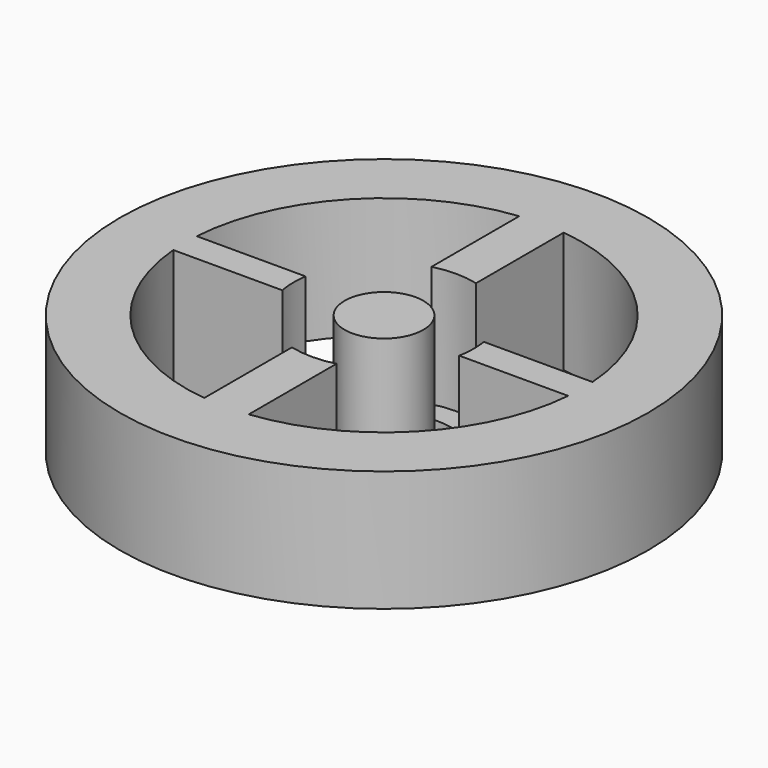
from build123d import *

# Parameters (mm, degrees)
F0_R     = 55.4446440976
F1_DEPTH = 25.4
F2_DEPTH = 25.4
F0_R_2   = 14.2471113664
F3_DEPTH = 7.112
F0_R_3   = 8.2640856971
F4_DEPTH = 25.4


# Not quite as in the source:
# - a feature names something its author has since deleted; it is built from what else it names


with BuildPart() as f1:
    # F0 (on Top) → F1 (new body)
    with BuildSketch(Plane.XY):
        Circle(F0_R)
        with BuildLine():
            ThreePointArc((4.6694431101, 41.3246424597), (30.0430645384, 28.7566348262), (41.4893209282, 2.8576252906))
            ThreePointArc((41.4893209282, 2.8576252906), (41.5630346864, 1.4296576644), (41.5876156251, 0))
            ThreePointArc((41.5876156251, 0), (41.551042786, -1.743736442), (41.4413885942, -3.4844059424))
            ThreePointArc((41.4413885942, -3.4844059424), (29.8248734287, -28.9828690496), (4.6694431101, -41.3246424597))
            ThreePointArc((4.6694431101, -41.3246424597), (0, -41.5876156251), (-4.6694431101, -41.3246424597))
            ThreePointArc((-4.6694431101, -41.3246424597), (-29.8248734287, -28.9828690496), (-41.4413885942, -3.4844059424))
            ThreePointArc((-41.4413885942, -3.4844059424), (-41.5859924727, -0.3674281517), (-41.496486252, 2.7516180913))
            ThreePointArc((-41.496486252, 2.7516180913), (-30.0797741132, 28.7182339757), (-4.6694431101, 41.3246424597))
            ThreePointArc((-4.6694431101, 41.3246424597), (0, 41.5876156251), (4.6694431101, 41.3246424597))
        make_face(mode=Mode.SUBTRACT)
    extrude(amount=F1_DEPTH)

    # F0 (on Top) → F2 (join)
    with BuildSketch(Plane.XY):
        Circle(F0_R)
        with BuildLine():
            ThreePointArc((4.6694431101, 41.3246424597), (30.0430645384, 28.7566348262), (41.4893209282, 2.8576252906))
            ThreePointArc((41.4893209282, 2.8576252906), (41.5630346864, 1.4296576644), (41.5876156251, 0))
            ThreePointArc((41.5876156251, 0), (41.551042786, -1.743736442), (41.4413885942, -3.4844059424))
            ThreePointArc((41.4413885942, -3.4844059424), (29.8248734287, -28.9828690496), (4.6694431101, -41.3246424597))
            ThreePointArc((4.6694431101, -41.3246424597), (0, -41.5876156251), (-4.6694431101, -41.3246424597))
            ThreePointArc((-4.6694431101, -41.3246424597), (-29.8248734287, -28.9828690496), (-41.4413885942, -3.4844059424))
            ThreePointArc((-41.4413885942, -3.4844059424), (-41.5859924727, -0.3674281517), (-41.496486252, 2.7516180913))
            ThreePointArc((-41.496486252, 2.7516180913), (-30.0797741132, 28.7182339757), (-4.6694431101, 41.3246424597))
            ThreePointArc((-4.6694431101, 41.3246424597), (0, 41.5876156251), (4.6694431101, 41.3246424597))
        make_face(mode=Mode.SUBTRACT)
        with BuildLine():
            ThreePointArc((-4.6694431101, 18.3096772012), (0, 18.895713222), (4.6694431101, 18.3096772012))
            Line((4.6694431101, 18.3096772012), (4.6694431101, 41.3246424597))
            ThreePointArc((4.6694431101, 41.3246424597), (0, 41.5876156251), (-4.6694431101, 41.3246424597))
            Line((-4.6694431101, 41.3246424597), (-4.6694431101, 18.3096772012))
        make_face()
        with BuildLine():
            ThreePointArc((-18.5716691064, -3.4844059424), (-18.8920611509, -0.3714884108), (-18.6942926063, 2.7516180913))
            Line((-18.6942926063, 2.7516180913), (-41.496486252, 2.7516180913))
            ThreePointArc((-41.496486252, 2.7516180913), (-41.5859924727, -0.3674281517), (-41.4413885942, -3.4844059424))
            Line((-41.4413885942, -3.4844059424), (-18.5716691064, -3.4844059424))
        make_face()
        with BuildLine():
            Line((4.6694431101, -41.3246424597), (4.6694431101, -18.3096772012))
            ThreePointArc((4.6694431101, -18.3096772012), (0, -18.895713222), (-4.6694431101, -18.3096772012))
            Line((-4.6694431101, -18.3096772012), (-4.6694431101, -41.3246424597))
            ThreePointArc((-4.6694431101, -41.3246424597), (0, -41.5876156251), (4.6694431101, -41.3246424597))
        make_face()
        with BuildLine():
            ThreePointArc((18.6783820463, 2.8576252906), (18.8413020883, 1.4329388631), (18.895713222, 0))
            ThreePointArc((18.895713222, 0), (18.8145277865, -1.7497206463), (18.5716691064, -3.4844059424))
            Line((18.5716691064, -3.4844059424), (41.4413885942, -3.4844059424))
            ThreePointArc((41.4413885942, -3.4844059424), (41.551042786, -1.743736442), (41.5876156251, 0))
            ThreePointArc((41.5876156251, 0), (41.5630346864, 1.4296576644), (41.4893209282, 2.8576252906))
            Line((41.4893209282, 2.8576252906), (18.6783820463, 2.8576252906))
        make_face()
    extrude(amount=F2_DEPTH)


with BuildPart() as f3:
    # F0 (on Top) → F3 (new body)
    with BuildSketch(Plane.XY):
        with BuildLine():
            Line((41.4413885942, -3.4844059424), (18.5716691064, -3.4844059424))
            ThreePointArc((18.5716691064, -3.4844059424), (13.7834861787, -12.925304133), (4.6694431101, -18.3096772012))
            Line((4.6694431101, -18.3096772012), (4.6694431101, -41.3246424597))
            ThreePointArc((4.6694431101, -41.3246424597), (29.8248734287, -28.9828690496), (41.4413885942, -3.4844059424))
        make_face()
        with BuildLine():
            ThreePointArc((18.5716691064, -3.4844059424), (18.8145277865, -1.7497206463), (18.895713222, 0))
            ThreePointArc((18.895713222, 0), (18.8413020883, 1.4329388631), (18.6783820463, 2.8576252906))
            ThreePointArc((18.6783820463, 2.8576252906), (13.9989896759, 12.6915824949), (4.6694431101, 18.3096772012))
            ThreePointArc((4.6694431101, 18.3096772012), (0, 18.895713222), (-4.6694431101, 18.3096772012))
            ThreePointArc((-4.6694431101, 18.3096772012), (-14.0349327563, 12.6518236115), (-18.6942926063, 2.7516180913))
            ThreePointArc((-18.6942926063, 2.7516180913), (-18.8920611509, -0.3714884108), (-18.5716691064, -3.4844059424))
            ThreePointArc((-18.5716691064, -3.4844059424), (-13.7834861787, -12.925304133), (-4.6694431101, -18.3096772012))
            ThreePointArc((-4.6694431101, -18.3096772012), (0, -18.895713222), (4.6694431101, -18.3096772012))
            ThreePointArc((4.6694431101, -18.3096772012), (13.7834861787, -12.925304133), (18.5716691064, -3.4844059424))
        make_face()
        Circle(F0_R_2, mode=Mode.SUBTRACT)
    extrude(amount=-F3_DEPTH)


with BuildPart() as f4:
    # F0 (on Top) → F4 (new body)
    with BuildSketch(Plane.XY):
        Circle(F0_R_3)
    extrude(amount=F4_DEPTH)


solid = Compound([f1.part, f3.part, f4.part])
